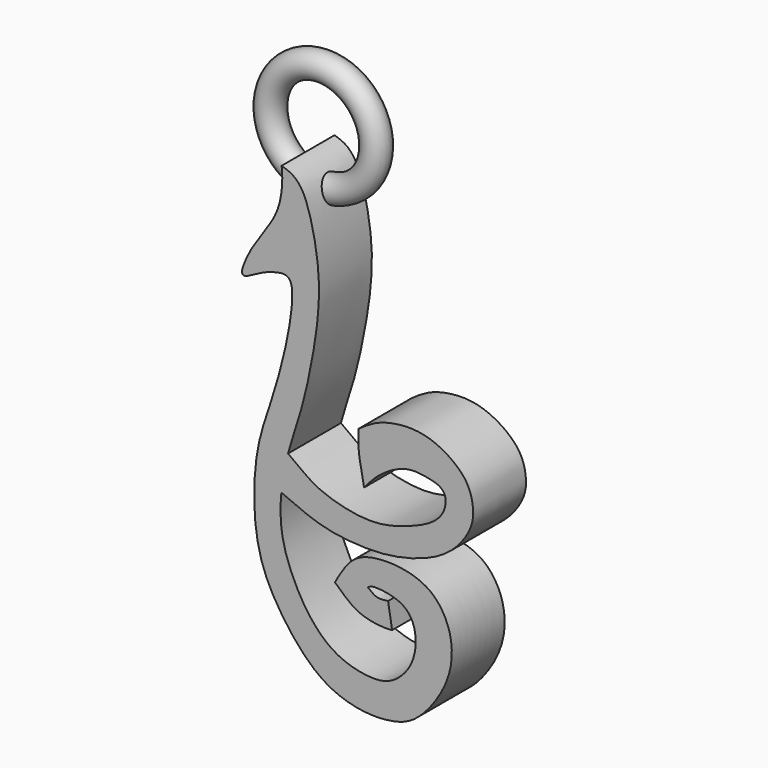
from build123d import *

# Parameters (mm, degrees)
F1_DEPTH = 2.5
F3_R     = 0.5


# Not quite as in the source:
# - a feature of the source that left no trace in its solid (it failed there, or was rolled back) is left out


with BuildPart() as f1:
    # F0 (on Front) → F1 (new body)
    with BuildSketch(Plane.XZ):
        with BuildLine():
            add(Edge.make_bspline(
                [(-1.7726288643, 7.4937217869), (-1.6254299601, 8.0591821532), (-1.2259084803, 9.0937926068), (-0.6903726988, 11.6788350146), (-0.4956453839, 13.8841811454), (-1.0152695585, 16.1613964449), (-1.4379335675, 16.7327132455), (-1.6815249154, 16.8951899193), (-2.0149676373, 17)],
                knots=[0.6118813074, 0.6118813074, 0.6118813074, 0.6118813074, 0.6791152276, 0.7616544482, 0.8411594877, 0.9182569305, 0.9584272588, 1, 1, 1, 1], degree=3))
            add(Edge.make_bspline(
                [(-2.0149676373, 17), (-1.9656486524, 16.5991608906), (-2.0114588148, 15.638178955), (-2.5972288493, 14.6742018365), (-3.1846931057, 13.9162458006), (-3.7513621292, 12.5920514079), (-2.8453175447, 13.1866538732), (-2.4694143434, 13.3088073892), (-1.9366620051, 13.4734573514), (-1.4881034834, 13.2359749948), (-1.7956456541, 11.0717155447), (-2.4204050211, 8.941146234), (-3.0810491803, 7.1441980968), (-3.1043298369, 4.1142228303), (-2.1940053499, 2.160518686), (-0.625221801, 0.2395167125), (1.0449483556, -0.2247052796), (2.131294575, -0.1794916378), (3.1477801786, 0.1133970244), (4.443024123, 1.8504527321), (4.4788204977, 3.5290687248), (3.7825767209, 4.6771348864), (2.7458134186, 5.0883628199), (1.6221184971, 5.1471587351), (0.5747804276, 4.8732090645), (0.1284792612, 4.0034242058), (0, 3.7819455476)],
                knots=[0, 0, 0, 0, 0.0420947907, 0.0802566863, 0.1187945715, 0.1539075331, 0.1831058829, 0.2087966534, 0.234772252, 0.2559542764, 0.3075833931, 0.3637408152, 0.4144060343, 0.47663661, 0.530860653, 0.5873323148, 0.6343508755, 0.6714924924, 0.7079538403, 0.7603100068, 0.8070283927, 0.847559745, 0.8851714736, 0.923667042, 0.9611044474, 1, 1, 1, 1], degree=3))
            add(Edge.make_bspline(
                [(0, 3.7819455476), (0.3034503376, 3.5129850477), (0.8420849821, 2.9324659818), (1.8680086693, 2.8558623561), (2.163980389, 2.8924297076)],
                knots=[0, 0, 0, 0, 0.4990166479, 1, 1, 1, 1], degree=3))
            Line((2.163980389, 2.8924297076), (2.0105831791, 3.8131189067))
            add(Edge.make_bspline(
                [(2.0105831791, 3.8131189067), (1.860844656, 3.7990672395), (1.5413491942, 3.7419433443), (1.3508246262, 3.95616265), (1.2435973622, 4.0179830976)],
                knots=[0, 0, 0, 0, 0.5205313518, 1, 1, 1, 1], degree=3))
            add(Edge.make_bspline(
                [(1.2435973622, 4.0179830976), (1.3501700931, 4.1035949668), (1.631709165, 4.1354313667), (2.7464380434, 3.9617793771), (3.145905977, 2.9843940382), (2.955080922, 1.9474735388), (2.3435356827, 1.2689088234), (1.6230076183, 0.9646589763), (0.1120392932, 1.2275194988), (-1.0332679252, 2.2888091644), (-1.8808878959, 3.9579854129), (-2.0930222374, 5.1211184808), (-2.0451943578, 5.9085021385), (-2.024621922, 6.1110760136)],
                knots=[0, 0, 0, 0, 0.0323452303, 0.0845305763, 0.1347650313, 0.1868339158, 0.234597264, 0.2788546909, 0.3404469835, 0.4047415731, 0.4742796506, 0.5390361644, 0.5610070323, 0.5610070323, 0.5610070323, 0.5610070323], degree=3))
            add(Edge.make_bspline(
                [(-2.024621922, 6.1110760136), (-1.9769857629, 6.5801425572), (-1.8840107015, 7.0658516555), (-1.7726288643, 7.4937217869)],
                knots=[0.5610070323, 0.5610070323, 0.5610070323, 0.5610070323, 0.6118813074, 0.6118813074, 0.6118813074, 0.6118813074], degree=3))
        make_face()
        with BuildLine():
            add(Edge.make_bspline(
                [(-1.7726288643, 7.4937217869), (-1.2903264637, 7.1664453174), (-0.8250569648, 6.6628062475), (1.3531357065, 6.0864609901), (2.7434397577, 6.5329820733), (3.6457822175, 6.8978478063), (4.1913376702, 7.4422927778), (4.2370326655, 8.252755275), (3.3907982746, 8.4411445967), (2.6469670978, 8.5138214387), (1.6502991777, 7.9469176244), (1.2875908468, 7.5138728), (1.1028246954, 7.2949388996)],
                knots=[0, 0, 0, 0, 0.1140170879, 0.2558121707, 0.3757039127, 0.4716311373, 0.5562058418, 0.6347035326, 0.7191185965, 0.8056711245, 0.9083541737, 1, 1, 1, 1], degree=3))
            add(Edge.make_bspline(
                [(-2.024621922, 6.1110760136), (-1.9769857629, 6.5801425572), (-1.8840107015, 7.0658516555), (-1.7726288643, 7.4937217869)],
                knots=[0.5610070323, 0.5610070323, 0.5610070323, 0.5610070323, 0.6118813074, 0.6118813074, 0.6118813074, 0.6118813074], degree=3))
            add(Edge.make_bspline(
                [(-2.024621922, 6.1110760136), (-1.5406921834, 5.9019148098), (-0.6474261488, 5.4936435422), (0.6623988204, 5.2939263008), (2.1537864474, 5.2830782014), (3.82887522, 5.772196202), (4.7247231772, 6.5215144714), (5.1872707557, 7.2835181637), (5.2639857262, 7.9013383638), (5.0677506424, 8.8495738657), (4.0030573425, 9.6440670056), (2.9079649402, 9.9279685288), (1.6367795247, 9.7121336655), (1.1301871754, 9.3529205926), (0.8967239992, 9.1873183846)],
                knots=[0, 0, 0, 0, 0.0955476014, 0.1839671446, 0.2791540132, 0.3812184505, 0.4647941, 0.5359291169, 0.5960535528, 0.6698373705, 0.7572428477, 0.8402643472, 0.9266589554, 1, 1, 1, 1], degree=3))
            add(Edge.make_bspline(
                [(1.1028246954, 7.2949388996), (1.0145498646, 7.7213109211), (0.8596424397, 8.469521836), (0.8855709781, 8.9714267083), (0.8967239992, 9.1873183846)],
                knots=[0, 0, 0, 0, 0.5698553884, 1, 1, 1, 1], degree=3))
        make_face()
    extrude(amount=F1_DEPTH)

    # F3 (on offset) → F4 (revolve)
    with BuildSketch(Plane.YZ.offset(-1.44)):
        with Locations((-1.25, 16)):
            Circle(F3_R)
    revolve(axis=Axis((-1.44, -0.1353690168, 18), (0, 1, 0)))


solid = f1.part
